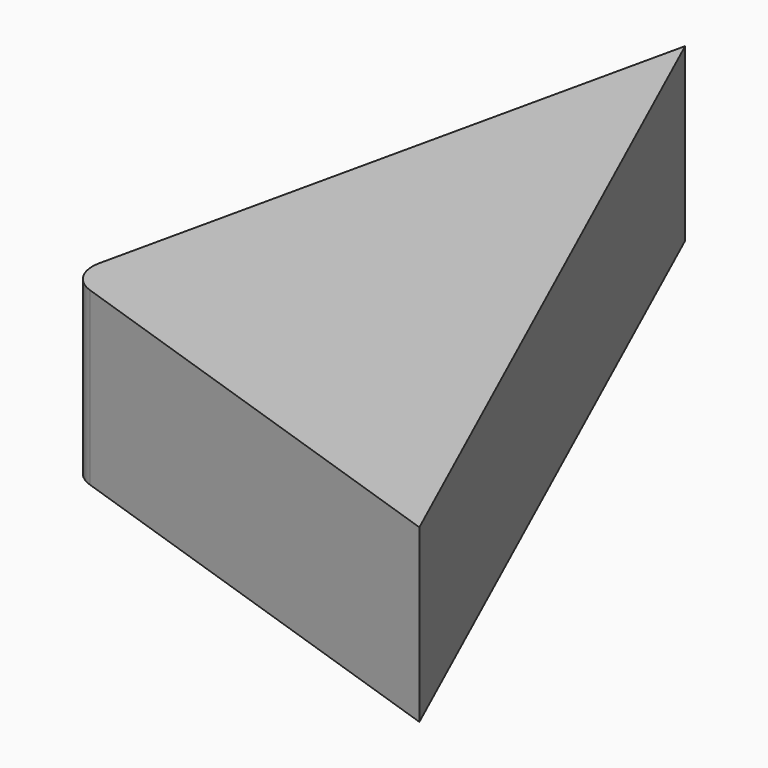
from build123d import *

# Parameters (mm, degrees)
F1_DEPTH = 25.4
F3_R     = 5.08


# Not quite as in the source:
# - a feature of the source that left no trace in its solid (it failed there, or was rolled back) is left out


with BuildPart() as f1:
    # F0 (on Top) → F1 (new body)
    with BuildSketch(Plane.XY):
        Polygon((-149.0168720484, -61.7396682501), (-77.7258127928, -85.825689137), (-129.0643811226, 27.6033654809), align=None)
    extrude(amount=F1_DEPTH)

    # F3
    f3_edges = [f1.edges().sort_by_distance(p)[0] for p in [
        (-149.016872, -61.739668, 12.7),
    ]]
    fillet(f3_edges, radius=F3_R)


solid = f1.part
